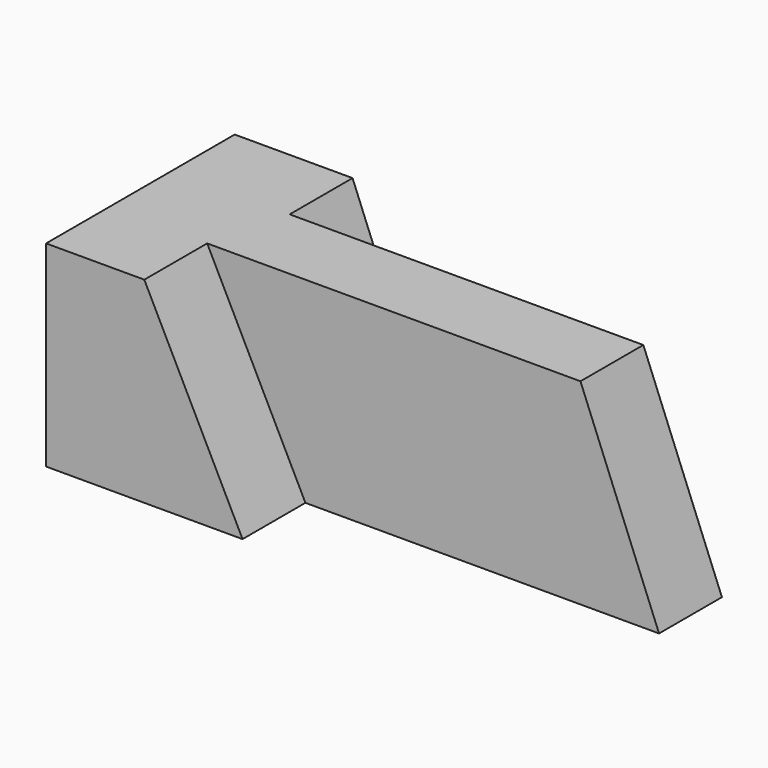
from build123d import *

# Parameters (mm, degrees)
F1_DEPTH = 31.75
F3_DEPTH = 25.4
F5_DEPTH = 12.7
F7_DEPTH = 12.7
F9_DEPTH = 12.7


# Not quite as in the source:
# - a length typed as a fraction of an inch, garbled in the dataset ("3 / 203.2 mm" for 3/8 in), is restored


with BuildPart() as f1:
    # F0 (on Top) → F1 (new body)
    with BuildSketch(Plane.XY):
        Polygon((-59.9109128669, -16.5989177401), (-91.6609128669, -16.5989177401), (-91.6609128669, -54.6989177401), (-59.9109128669, -54.6989177401), (-59.9109128669, -41.9989177401), (-2.7609128669, -41.9989177401), (-2.7609128669, -29.2989177401), (-59.9109128669, -29.2989177401), align=None)
    extrude(amount=F1_DEPTH)

    # F2 (on face) → F3 (cut)
    with BuildSketch(Plane.XZ.offset(54.6989177401)):
        Polygon((-74.4201987982, 31.75), (-59.9109128669, 0), (-59.9109128669, 31.75), align=None)
    extrude(amount=F3_DEPTH, mode=Mode.SUBTRACT)

    # F4 (on face) → F5 (cut)
    with BuildSketch(Plane.XZ.offset(54.6989177401)):
        Polygon((-75.7859128669, 31.75), (-59.9109128669, 0), (-46.3341996074, 12.059702538), (-46.3341996074, 45.9536202252), (-62.0433166623, 45.9536202252), align=None)
    extrude(amount=-F5_DEPTH, mode=Mode.SUBTRACT)

    # F6 (on face) → F7 (cut)
    with BuildSketch(Plane(origin=(0, -16.5989177401, 0), x_dir=(-1, 0, 0), z_dir=(0, 1, 0))):
        Polygon((59.9109128669, 0), (72.6109128669, 31.75), (59.9109128669, 31.75), align=None)
    extrude(amount=-F7_DEPTH, mode=Mode.SUBTRACT)

    # F8 (on face) → F9 (cut)
    with BuildSketch(Plane.XZ.offset(41.9989177401)):
        Polygon((-15.4609128669, 31.75), (-2.7609128669, 0), (-2.7609128669, 31.75), align=None)
    extrude(amount=-F9_DEPTH, mode=Mode.SUBTRACT)


solid = f1.part
